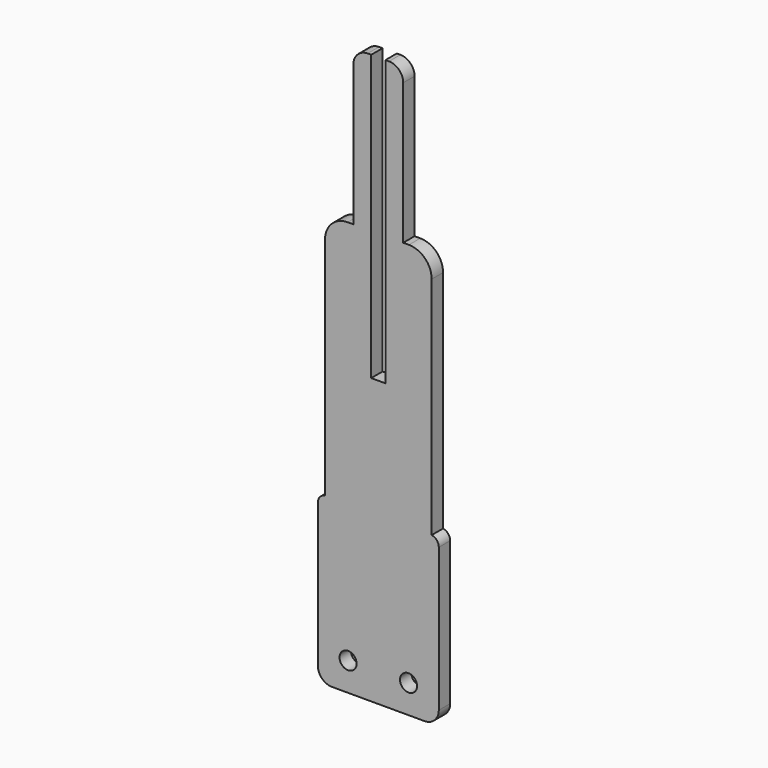
from build123d import *

# Parameters (mm, degrees)
F0_R        = 3.81
F1_DEPTH    = 3.175
F2_R        = 10.16
F3_R        = 6.35
F4_T1_DEPTH = 25.1335533113
F5_R        = 6.35


# Not quite as in the source:
# - a fillet or chamfer that OpenCascade refuses, or shapes differently, is made with other operations: its cross-section is extruded or revolved along the edge and cut away or added


with BuildPart() as f1:
    # F0 (on Front) → F1 (new body, symmetric)
    with BuildSketch(Plane.XZ):
        Polygon((-49.1121449284, -23.3316957779), (-52.2871449284, -23.3316957779), (-52.2871449284, -97.4421674833), (1.6878550716, -97.4421674833), (1.6878550716, -23.3316957779), (-1.4871449284, -23.3316957779), (-1.4871449284, 87.3682325167), (-14.1871449284, 87.3682325167), (-14.1871449284, 156.5578325167), (-22.1246449284, 156.5578325167), (-22.1246449284, 29.5578325167), (-28.4746449284, 29.5578325167), (-28.4746449284, 156.5578325167), (-36.4121449284, 156.5578325167), (-36.4121449284, 87.3682325167), (-49.1121449284, 87.3682325167), align=None)
        with Locations((-38.7933949284, -84.7421674833)):
            Circle(F0_R, mode=Mode.SUBTRACT)
        with Locations((-11.8185949284, -84.7421674833)):
            Circle(F0_R, mode=Mode.SUBTRACT)
    extrude(amount=F1_DEPTH, both=True)

    # F2
    f2_edges = [f1.edges().sort_by_distance(p)[0] for p in [
        (-1.487145, 0, 87.368233),
        (-49.112145, 0, 87.368233),
    ]]
    fillet(f2_edges, radius=F2_R)

    # F3
    f3_edges = [f1.edges().sort_by_distance(p)[0] for p in [
        (-14.187145, 0, 156.557833),
        (-36.412145, 0, 156.557833),
    ]]
    fillet(f3_edges, radius=F3_R)

    # F4: fillet of radius 3.81 on 2 edges, made by hand

    # F4_s2 → F4_t1 (cut)
    with BuildSketch(Plane.XZ.offset(-12.5667766557)):
        with BuildLine():
            ThreePointArc((-49.1121449284, -23.3316957779), (-51.3870804947, -24.6290620154), (-52.2871449284, -27.0884064402))
            Line((-52.2871449284, -27.0884064402), (-52.2871449284, -23.3316957779))
            Line((-52.2871449284, -23.3316957779), (-49.1121449284, -23.3316957779))
        make_face()
        with BuildLine():
            ThreePointArc((1.6878550716, -27.0884064402), (0.7877906379, -24.6290620154), (-1.4871449284, -23.3316957779))
            Line((-1.4871449284, -23.3316957779), (1.6878550716, -23.3316957779))
            Line((1.6878550716, -23.3316957779), (1.6878550716, -27.0884064402))
        make_face()
    extrude(amount=F4_T1_DEPTH, mode=Mode.SUBTRACT)

    # F5
    f5_edges = [f1.edges().sort_by_distance(p)[0] for p in [
        (-52.287145, 0, -97.442167),
        (1.687855, 0, -97.442167),
    ]]
    fillet(f5_edges, radius=F5_R)


solid = f1.part
